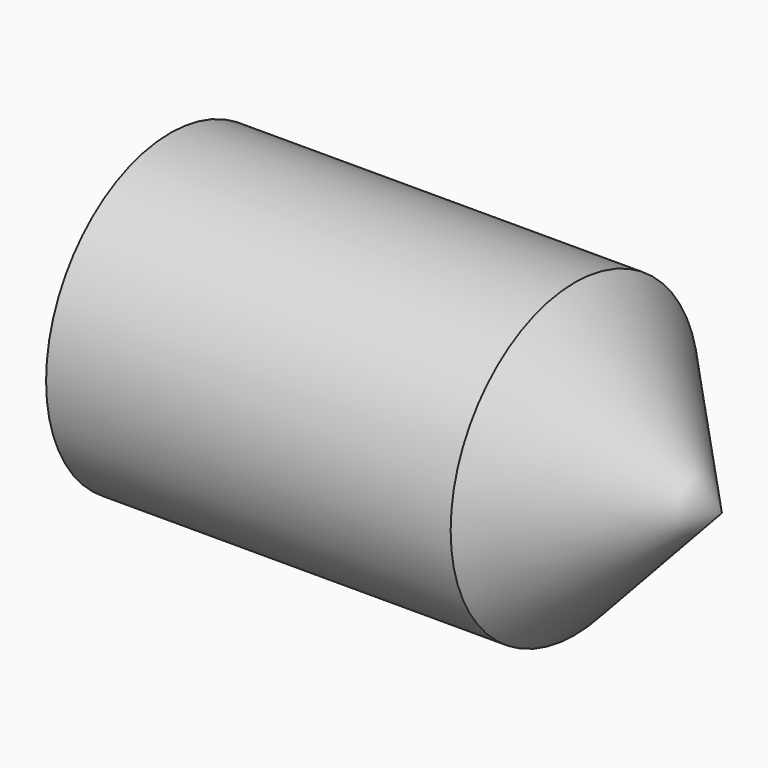
from build123d import *


# Not quite as in the source:
# - the program builds the solid bodies; features that only make, move or delete a surface that nothing else refers to are left out


with BuildPart() as f3:
    # F2 (on Front) → F3 (revolve)
    with BuildSketch(Plane.XZ):
        Polygon((-12.7874528989, 0), (-16.660457477, 4.0856003761), (-27.3112170398, 4.0856003761), (-27.3112170398, 0), align=None)
    revolve(axis=Axis((27.1737959197, 0, 0), (-1, 0, 0)))


solid = f3.part
